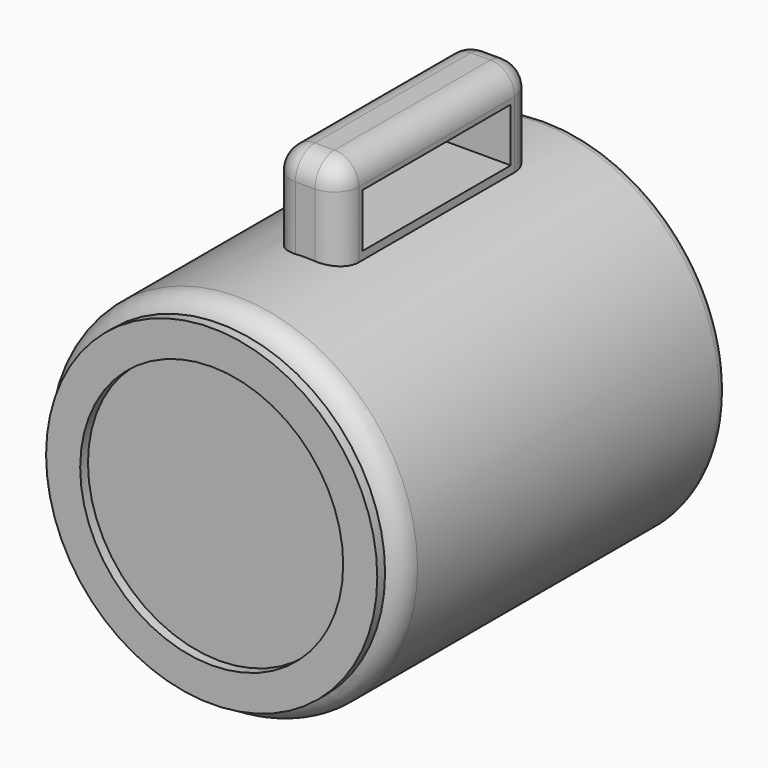
from build123d import *

# Parameters (mm, degrees)
F2_R     = 2
F5_W     = 7
F5_H     = 50
F6_DEPTH = 20
F8_R     = 5
F7_W     = 38
F7_H     = 11
F9_DEPTH = 25


# Not quite as in the source:
# - a fillet or chamfer that OpenCascade refuses, or shapes differently, is made with other operations: its cross-section is extruded or revolved along the edge and cut away or added
# - two fillets or chamfers of one size are made in one step


with BuildPart() as f1:
    # F0 (on Top) → F1 (revolve)
    with BuildSketch(Plane.XY):
        Polygon((0, -7), (0, 0), (-30, 0), (-30, 77), (-37, 77), (-37, -7), (-34, -7), (-34, -9), (-27, -9), (-27, -7), align=None)
    revolve(axis=Axis((0, 38.5, 0), (0, 1, 0)))

    # F2
    f2_edges = [f1.edges().sort_by_distance(p)[0] for p in [
        (37, 77, 0),
        (30, 77, 0),
    ]]
    fillet(f2_edges, radius=F2_R)

    # F3: fillet of radius 5 on 1 edges, made by hand

    # F3_s1 → F3_t2 (revolve, cut)
    with BuildSketch(Plane.XY):
        with BuildLine():
            ThreePointArc((-37, -2.417424305), (-36.1833001327, -5.1560370926), (-34, -7))
            Line((-34, -7), (-37, -7))
            Line((-37, -7), (-37, -2.417424305))
        make_face()
    revolve(axis=Axis((0, -7, 0), (0, 1, 0)), mode=Mode.SUBTRACT)

    # F5 (on offset) → F6 (join)
    with BuildSketch(Plane.XY.offset(35)):
        with Locations((-3.5, 40)):
            Rectangle(F5_W, F5_H)
        with Locations((3.5, 40)):
            Rectangle(F5_W, F5_H)
    extrude(amount=F6_DEPTH)

    # F8
    f8_edges = [f1.edges().sort_by_distance(p)[0] for p in [
        (0, 65, 55),
        (0, 15, 55),
        (7, 15, 45.665902),
        (-7, 15, 45.665902),
        (-7, 40, 55),
        (-7, 65, 45.665902),
        (7, 65, 45.665902),
        (7, 40, 55),
    ]]
    fillet(f8_edges, radius=F8_R)

    # F7 (on face) → F9 (cut)
    with BuildSketch(Plane.YZ.offset(7)):
        with Locations((40, 43.5)):
            Rectangle(F7_W, F7_H)
    extrude(amount=-F9_DEPTH, mode=Mode.SUBTRACT)


solid = f1.part
